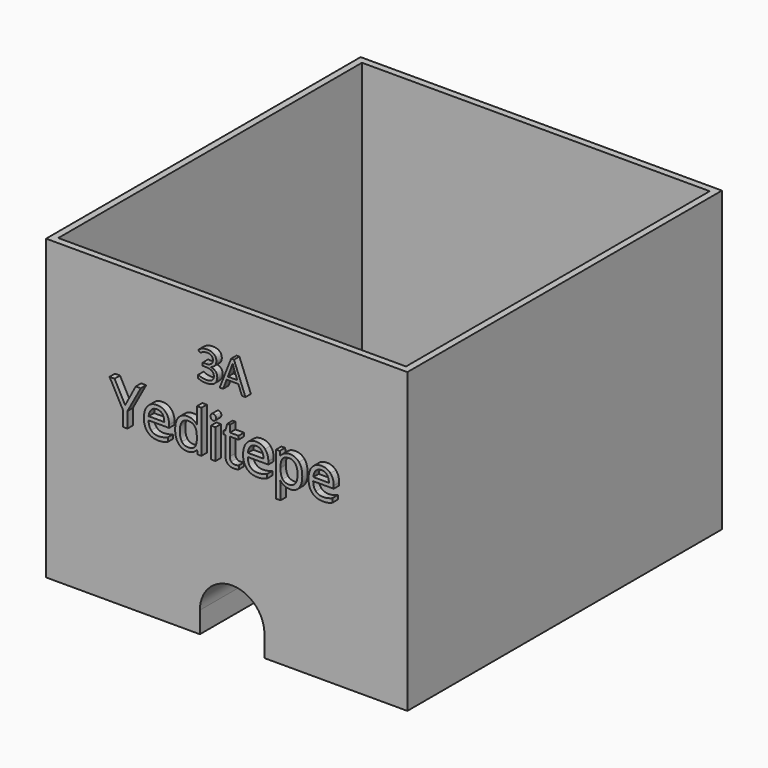
from build123d import *

# Parameters (mm, degrees)
F0_W         = 53.3
F0_H         = 44
F2_DEPTH     = 58
F3_DEPTH     = 58.001
F4_T         = -1
F5_W         = 0.6667008056
F5_H         = 4.399711482
F6_DEPTH     = 1
F7_TEXT_SIZE = 6.0143104444
F8_DEPTH     = 1


# Not quite as in the source:
# - a feature names something its author has since deleted; it is built from what else it names
# - Text() gives the source's letters only with a copy of the font that has no kerning and outlines rounded to 1/6400 em; it was checked with that copy


with BuildPart() as f2:
    # F0 (on Front) → F2 (new body)
    with BuildSketch(Plane.XZ):
        with Locations((26.65, 22)):
            Rectangle(F0_W, F0_H)
    extrude(amount=-F2_DEPTH)

    # F1 (on face) → F3 (cut, through all)
    with BuildSketch(Plane.XZ):
        with BuildLine():
            Line((22.69, 0), (27.45, 0))
            Line((27.45, 0), (32.21, 0))
            Line((32.21, 0), (32.21, 3.132))
            ThreePointArc((32.21, 3.132), (27.45, 7.892), (22.69, 3.132))
            Line((22.69, 3.132), (22.69, 0))
        make_face()
    extrude(amount=-F3_DEPTH, mode=Mode.SUBTRACT)

    # F4
    f4_openings = [f2.faces().sort_by_distance(p)[0] for p in [
        (26.65, 29, 44),
    ]]
    offset(amount=F4_T, openings=f4_openings)


with BuildPart() as f6:
    # F5 (on face) → F6 (new body)
    with BuildSketch(Plane.XZ):
        Polygon((14.0276988229, 29.7714103198), (12.4630714988, 26.836128353), (10.908720873, 29.7714103198), (10.1623756552, 29.7714103198), (12.1175175167, 26.1463049761), (12.1175175167, 23.9021309735), (12.8073408936, 23.9021309735), (12.8073408936, 26.1784196585), (14.7663365169, 29.7714103198), align=None)
        with BuildLine():
            add(Edge.make_bspline(
                [(17.3316573431, 23.8212019739), (16.3566555869, 23.8212019739), (15.7920794712, 24.4159658911)],
                knots=[0, 0, 0, 1, 1, 1], degree=2))
            add(Edge.make_bspline(
                [(18.0921330212, 23.8880005132), (17.7774091341, 23.8212019739), (17.3316573431, 23.8212019739)],
                knots=[0, 0, 0, 1, 1, 1], degree=2))
            add(Edge.make_bspline(
                [(18.760118414, 24.1063803532), (18.4068569082, 23.9547990525), (18.0921330212, 23.8880005132)],
                knots=[0, 0, 0, 1, 1, 1], degree=2))
            Line((18.760118414, 24.1063803532), (18.760118414, 24.7011442703))
            add(Edge.make_bspline(
                [(17.3560645017, 24.4044046054), (18.0664412753, 24.4044046054), (18.760118414, 24.7011442703)],
                knots=[0, 0, 0, 1, 1, 1], degree=2))
            add(Edge.make_bspline(
                [(16.3104104443, 24.8058381348), (16.6816561723, 24.4044046054), (17.3560645017, 24.4044046054)],
                knots=[0, 0, 0, 1, 1, 1], degree=2))
            add(Edge.make_bspline(
                [(15.9186113197, 25.9818778025), (15.9391647164, 25.2072716642), (16.3104104443, 24.8058381348)],
                knots=[0, 0, 0, 1, 1, 1], degree=2))
            Line((15.9186113197, 25.9818778025), (18.9489527463, 25.9818778025))
            Line((18.9489527463, 25.9818778025), (18.9489527463, 26.4032224349))
            add(Edge.make_bspline(
                [(18.467232511, 27.838748736), (18.9489527463, 27.294726017), (18.9489527463, 26.4032224349)],
                knots=[0, 0, 0, 1, 1, 1], degree=2))
            add(Edge.make_bspline(
                [(17.1595226457, 28.382771455), (17.9855122757, 28.382771455), (18.467232511, 27.838748736)],
                knots=[0, 0, 0, 1, 1, 1], degree=2))
            add(Edge.make_bspline(
                [(15.7516149715, 27.7565351492), (16.2757265874, 28.382771455), (17.1595226457, 28.382771455)],
                knots=[0, 0, 0, 1, 1, 1], degree=2))
            add(Edge.make_bspline(
                [(15.2275033555, 26.0653759766), (15.2275033555, 27.1302988433), (15.7516149715, 27.7565351492)],
                knots=[0, 0, 0, 1, 1, 1], degree=2))
            add(Edge.make_bspline(
                [(15.7920794712, 24.4159658911), (15.2275033555, 25.0107298082), (15.2275033555, 26.0653759766)],
                knots=[0, 0, 0, 1, 1, 1], degree=2))
        make_face()
        with BuildLine():
            add(Edge.make_bspline(
                [(17.1505305346, 27.8239759821), (16.6212805695, 27.8239759821), (16.3059143888, 27.4790642936)],
                knots=[0, 0, 0, 1, 1, 1], degree=2))
            add(Edge.make_bspline(
                [(17.954039887, 27.4886986984), (17.6733575633, 27.8239759821), (17.1505305346, 27.8239759821)],
                knots=[0, 0, 0, 1, 1, 1], degree=2))
            add(Edge.make_bspline(
                [(18.2347222108, 26.5239736405), (18.2347222108, 27.1534214146), (17.954039887, 27.4886986984)],
                knots=[0, 0, 0, 1, 1, 1], degree=2))
            Line((18.2347222108, 26.5239736405), (15.9340263672, 26.5239736405))
            add(Edge.make_bspline(
                [(16.3059143888, 27.4790642936), (15.9905482081, 27.1341526052), (15.9340263672, 26.5239736405)],
                knots=[0, 0, 0, 1, 1, 1], degree=2))
        make_face(mode=Mode.SUBTRACT)
        with BuildLine():
            Line((23.0442170396, 24.4917565414), (23.0801854838, 24.4917565414))
            Line((23.0801854838, 24.4917565414), (23.1688220071, 23.9021309735))
            Line((23.1688220071, 23.9021309735), (23.7109178452, 23.9021309735))
            Line((23.7109178452, 23.9021309735), (23.7109178452, 30.1490789843))
            Line((23.7109178452, 30.1490789843), (23.0442170396, 30.1490789843))
            Line((23.0442170396, 30.1490789843), (23.0442170396, 28.3583642964))
            Line((23.0442170396, 28.3583642964), (23.0609166744, 28.0487787585))
            Line((23.0609166744, 28.0487787585), (23.0891775949, 27.7314856969))
            Line((23.0891775949, 27.7314856969), (23.0365095158, 27.7314856969))
            add(Edge.make_bspline(
                [(21.6632856985, 28.382771455), (22.5586430425, 28.382771455), (23.0365095158, 27.7314856969)],
                knots=[0, 0, 0, 1, 1, 1], degree=2))
            add(Edge.make_bspline(
                [(20.3221765636, 27.7803000141), (20.8038967988, 28.382771455), (21.6632856985, 28.382771455)],
                knots=[0, 0, 0, 1, 1, 1], degree=2))
            add(Edge.make_bspline(
                [(19.8404563283, 26.0897831352), (19.8404563283, 27.1778285732), (20.3221765636, 27.7803000141)],
                knots=[0, 0, 0, 1, 1, 1], degree=2))
            add(Edge.make_bspline(
                [(20.3202496826, 24.4114698355), (19.8404563283, 25.0017376971), (19.8404563283, 26.0897831352)],
                knots=[0, 0, 0, 1, 1, 1], degree=2))
            add(Edge.make_bspline(
                [(21.6632856985, 23.8212019739), (20.8000430369, 23.8212019739), (20.3202496826, 24.4114698355)],
                knots=[0, 0, 0, 1, 1, 1], degree=2))
            add(Edge.make_bspline(
                [(23.0442170396, 24.4917565414), (22.583050201, 23.8212019739), (21.6632856985, 23.8212019739)],
                knots=[0, 0, 0, 1, 1, 1], degree=2))
        make_face()
        with BuildLine():
            add(Edge.make_bspline(
                [(21.7480684599, 24.3799974468), (22.4301843131, 24.3799974468), (22.7372006763, 24.7512431748)],
                knots=[0, 0, 0, 1, 1, 1], degree=2))
            add(Edge.make_bspline(
                [(20.8405075367, 24.8096918967), (21.1494507809, 24.3799974468), (21.7480684599, 24.3799974468)],
                knots=[0, 0, 0, 1, 1, 1], degree=2))
            add(Edge.make_bspline(
                [(20.5315642925, 26.0820756114), (20.5315642925, 25.2393863465), (20.8405075367, 24.8096918967)],
                knots=[0, 0, 0, 1, 1, 1], degree=2))
            add(Edge.make_bspline(
                [(20.8424344176, 27.3685897864), (20.5315642925, 26.9132035906), (20.5315642925, 26.0820756114)],
                knots=[0, 0, 0, 1, 1, 1], degree=2))
            add(Edge.make_bspline(
                [(21.7403609362, 27.8239759821), (21.1533045428, 27.8239759821), (20.8424344176, 27.3685897864)],
                knots=[0, 0, 0, 1, 1, 1], degree=2))
            add(Edge.make_bspline(
                [(22.7333469144, 27.4244693337), (22.4224767893, 27.8239759821), (21.7403609362, 27.8239759821)],
                knots=[0, 0, 0, 1, 1, 1], degree=2))
            add(Edge.make_bspline(
                [(23.0442170396, 26.0897831352), (23.0442170396, 27.0249626852), (22.7333469144, 27.4244693337)],
                knots=[0, 0, 0, 1, 1, 1], degree=2))
            Line((23.0442170396, 26.0897831352), (23.0442170396, 25.9497631201))
            add(Edge.make_bspline(
                [(22.7372006763, 24.7512431748), (23.0442170396, 25.1224889028), (23.0442170396, 25.9497631201)],
                knots=[0, 0, 0, 1, 1, 1], degree=2))
        make_face(mode=Mode.SUBTRACT)
        with Locations((25.4573142714, 26.1019867145)):
            Rectangle(F5_W, F5_H)
        with BuildLine():
            add(Edge.make_bspline(
                [(25.0674420277, 29.4939394643), (25.0674420277, 29.7225960026), (25.1798434159, 29.8292167481)],
                knots=[0, 0, 0, 1, 1, 1], degree=2))
            add(Edge.make_bspline(
                [(25.1798434159, 29.1586621806), (25.0674420277, 29.2691366879), (25.0674420277, 29.4939394643)],
                knots=[0, 0, 0, 1, 1, 1], degree=2))
            add(Edge.make_bspline(
                [(25.4618103269, 29.0481876733), (25.2922448041, 29.0481876733), (25.1798434159, 29.1586621806)],
                knots=[0, 0, 0, 1, 1, 1], degree=2))
            add(Edge.make_bspline(
                [(25.7386388888, 29.1586621806), (25.6223837387, 29.0481876733), (25.4618103269, 29.0481876733)],
                knots=[0, 0, 0, 1, 1, 1], degree=2))
            add(Edge.make_bspline(
                [(25.8548940389, 29.4939394643), (25.8548940389, 29.2691366879), (25.7386388888, 29.1586621806)],
                knots=[0, 0, 0, 1, 1, 1], degree=2))
            add(Edge.make_bspline(
                [(25.7386388888, 29.8272898671), (25.8548940389, 29.7187422408), (25.8548940389, 29.4939394643)],
                knots=[0, 0, 0, 1, 1, 1], degree=2))
            add(Edge.make_bspline(
                [(25.4618103269, 29.9358374935), (25.6223837387, 29.9358374935), (25.7386388888, 29.8272898671)],
                knots=[0, 0, 0, 1, 1, 1], degree=2))
            add(Edge.make_bspline(
                [(25.1798434159, 29.8292167481), (25.2922448041, 29.9358374935), (25.4618103269, 29.9358374935)],
                knots=[0, 0, 0, 1, 1, 1], degree=2))
        make_face()
        with BuildLine():
            Line((26.9984875229, 28.2710156541), (27.0092743154, 27.784153776))
            Line((27.0092743154, 27.784153776), (27.2525250148, 27.784153776))
            Line((27.2525250148, 27.784153776), (27.2525250148, 25.1661648708))
            add(Edge.make_bspline(
                [(28.5281201978, 23.8212019739), (27.2525250148, 23.8212019739), (27.2525250148, 25.1661648708)],
                knots=[0, 0, 0, 1, 1, 1], degree=2))
            add(Edge.make_bspline(
                [(28.9083580368, 23.8558858309), (28.6976857206, 23.8212019739), (28.5281201978, 23.8212019739)],
                knots=[0, 0, 0, 1, 1, 1], degree=2))
            add(Edge.make_bspline(
                [(29.2269356857, 23.9419531796), (29.119030353, 23.8905696878), (28.9083580368, 23.8558858309)],
                knots=[0, 0, 0, 1, 1, 1], degree=2))
            Line((29.2269356857, 23.9419531796), (29.2269356857, 24.4519343353))
            add(Edge.make_bspline(
                [(28.966164465, 24.3979816689), (29.1305916387, 24.4236734148), (29.2269356857, 24.4519343353)],
                knots=[0, 0, 0, 1, 1, 1], degree=2))
            add(Edge.make_bspline(
                [(28.6244642448, 24.3722899231), (28.8017372914, 24.3722899231), (28.966164465, 24.3979816689)],
                knots=[0, 0, 0, 1, 1, 1], degree=2))
            add(Edge.make_bspline(
                [(28.1067755653, 24.5848891202), (28.2956098975, 24.3722899231), (28.6244642448, 24.3722899231)],
                knots=[0, 0, 0, 1, 1, 1], degree=2))
            add(Edge.make_bspline(
                [(27.9179412331, 25.1944257912), (27.9179412331, 24.7974883174), (28.1067755653, 24.5848891202)],
                knots=[0, 0, 0, 1, 1, 1], degree=2))
            Line((27.9179412331, 25.1944257912), (27.9179412331, 27.784153776))
            Line((27.9179412331, 27.784153776), (29.1948210034, 27.784153776))
            Line((29.1948210034, 27.784153776), (29.1948210034, 28.3018424555))
            Line((29.1948210034, 28.3018424555), (27.9179412331, 28.3018424555))
            Line((27.9179412331, 28.3018424555), (27.9179412331, 29.3218047669))
            Line((27.9179412331, 29.3218047669), (27.5325650449, 29.3218047669))
            Line((27.5325650449, 29.3218047669), (27.2525250148, 28.382771455))
            Line((27.2525250148, 28.382771455), (26.9984875229, 28.2710156541))
        make_face()
        with BuildLine():
            add(Edge.make_bspline(
                [(31.9643912093, 23.8212019739), (30.9893894531, 23.8212019739), (30.4248133374, 24.4159658911)],
                knots=[0, 0, 0, 1, 1, 1], degree=2))
            add(Edge.make_bspline(
                [(32.7248668873, 23.8880005132), (32.4101430003, 23.8212019739), (31.9643912093, 23.8212019739)],
                knots=[0, 0, 0, 1, 1, 1], degree=2))
            add(Edge.make_bspline(
                [(33.3928522802, 24.1063803532), (33.0395907744, 23.9547990525), (32.7248668873, 23.8880005132)],
                knots=[0, 0, 0, 1, 1, 1], degree=2))
            Line((33.3928522802, 24.1063803532), (33.3928522802, 24.7011442703))
            add(Edge.make_bspline(
                [(31.9887983678, 24.4044046054), (32.6991751414, 24.4044046054), (33.3928522802, 24.7011442703)],
                knots=[0, 0, 0, 1, 1, 1], degree=2))
            add(Edge.make_bspline(
                [(30.9431443105, 24.8058381348), (31.3143900385, 24.4044046054), (31.9887983678, 24.4044046054)],
                knots=[0, 0, 0, 1, 1, 1], degree=2))
            add(Edge.make_bspline(
                [(30.5513451858, 25.9818778025), (30.5718985825, 25.2072716642), (30.9431443105, 24.8058381348)],
                knots=[0, 0, 0, 1, 1, 1], degree=2))
            Line((30.5513451858, 25.9818778025), (33.5816866124, 25.9818778025))
            Line((33.5816866124, 25.9818778025), (33.5816866124, 26.4032224349))
            add(Edge.make_bspline(
                [(33.0999663772, 27.838748736), (33.5816866124, 27.294726017), (33.5816866124, 26.4032224349)],
                knots=[0, 0, 0, 1, 1, 1], degree=2))
            add(Edge.make_bspline(
                [(31.7922565119, 28.382771455), (32.6182461419, 28.382771455), (33.0999663772, 27.838748736)],
                knots=[0, 0, 0, 1, 1, 1], degree=2))
            add(Edge.make_bspline(
                [(30.3843488376, 27.7565351492), (30.9084604536, 28.382771455), (31.7922565119, 28.382771455)],
                knots=[0, 0, 0, 1, 1, 1], degree=2))
            add(Edge.make_bspline(
                [(29.8602372217, 26.0653759766), (29.8602372217, 27.1302988433), (30.3843488376, 27.7565351492)],
                knots=[0, 0, 0, 1, 1, 1], degree=2))
            add(Edge.make_bspline(
                [(30.4248133374, 24.4159658911), (29.8602372217, 25.0107298082), (29.8602372217, 26.0653759766)],
                knots=[0, 0, 0, 1, 1, 1], degree=2))
        make_face()
        with BuildLine():
            add(Edge.make_bspline(
                [(31.7832644008, 27.8239759821), (31.2540144357, 27.8239759821), (30.938648255, 27.4790642936)],
                knots=[0, 0, 0, 1, 1, 1], degree=2))
            add(Edge.make_bspline(
                [(32.5867737532, 27.4886986984), (32.3060914295, 27.8239759821), (31.7832644008, 27.8239759821)],
                knots=[0, 0, 0, 1, 1, 1], degree=2))
            add(Edge.make_bspline(
                [(32.867456077, 26.5239736405), (32.867456077, 27.1534214146), (32.5867737532, 27.4886986984)],
                knots=[0, 0, 0, 1, 1, 1], degree=2))
            Line((32.867456077, 26.5239736405), (30.5667602334, 26.5239736405))
            add(Edge.make_bspline(
                [(30.938648255, 27.4790642936), (30.6232820743, 27.1341526052), (30.5667602334, 26.5239736405)],
                knots=[0, 0, 0, 1, 1, 1], degree=2))
        make_face(mode=Mode.SUBTRACT)
        with BuildLine():
            add(Edge.make_bspline(
                [(36.7661785143, 23.8212019739), (36.3358417708, 23.8212019739), (35.980653384, 23.9798485047)],
                knots=[0, 0, 0, 1, 1, 1], degree=2))
            add(Edge.make_bspline(
                [(38.1092145302, 24.4217465339), (37.625567414, 23.8212019739), (36.7661785143, 23.8212019739)],
                knots=[0, 0, 0, 1, 1, 1], degree=2))
            add(Edge.make_bspline(
                [(38.5928616464, 26.10648277), (38.5928616464, 25.0222910938), (38.1092145302, 24.4217465339)],
                knots=[0, 0, 0, 1, 1, 1], degree=2))
            add(Edge.make_bspline(
                [(38.116922054, 27.784153776), (38.5928616464, 27.185536097), (38.5928616464, 26.10648277)],
                knots=[0, 0, 0, 1, 1, 1], degree=2))
            add(Edge.make_bspline(
                [(36.7661785143, 28.382771455), (37.6409824615, 28.382771455), (38.116922054, 27.784153776)],
                knots=[0, 0, 0, 1, 1, 1], degree=2))
            add(Edge.make_bspline(
                [(35.9832225586, 28.2221980432), (36.3242804852, 28.382771455), (36.7661785143, 28.382771455)],
                knots=[0, 0, 0, 1, 1, 1], degree=2))
            add(Edge.make_bspline(
                [(35.3852471732, 27.6993710146), (35.642164632, 28.0616246315), (35.9832225586, 28.2221980432)],
                knots=[0, 0, 0, 1, 1, 1], degree=2))
            Line((35.3852471732, 27.6993710146), (35.3531324909, 27.6993710146))
            Line((35.3531324909, 27.6993710146), (35.2606422057, 28.3018424555))
            Line((35.2606422057, 28.3018424555), (34.7185463676, 28.3018424555))
            Line((34.7185463676, 28.3018424555), (34.7185463676, 21.9264357153))
            Line((34.7185463676, 21.9264357153), (35.3852471732, 21.9264357153))
            Line((35.3852471732, 21.9264357153), (35.3852471732, 23.7377037998))
            add(Edge.make_bspline(
                [(35.3364328561, 24.4686339701), (35.3852471732, 24.0832577819), (35.3852471732, 23.7377037998)],
                knots=[0, 0, 0, 1, 1, 1], degree=2))
            Line((35.3364328561, 24.4686339701), (35.3852471732, 24.4686339701))
            add(Edge.make_bspline(
                [(35.980653384, 23.9798485047), (35.6254649972, 24.1384950356), (35.3852471732, 24.4686339701)],
                knots=[0, 0, 0, 1, 1, 1], degree=2))
        make_face()
        with BuildLine():
            add(Edge.make_bspline(
                [(36.6698344672, 27.8162684583), (35.9954261379, 27.8162684583), (35.6941904174, 27.4430958494)],
                knots=[0, 0, 0, 1, 1, 1], degree=2))
            add(Edge.make_bspline(
                [(37.5786799778, 27.3769396038), (37.2556062733, 27.8162684583), (36.6698344672, 27.8162684583)],
                knots=[0, 0, 0, 1, 1, 1], degree=2))
            add(Edge.make_bspline(
                [(37.9017536822, 26.1141902938), (37.9017536822, 26.9376107492), (37.5786799778, 27.3769396038)],
                knots=[0, 0, 0, 1, 1, 1], degree=2))
            add(Edge.make_bspline(
                [(37.5786799778, 24.841806579), (37.9017536822, 25.3036157112), (37.9017536822, 26.1141902938)],
                knots=[0, 0, 0, 1, 1, 1], degree=2))
            add(Edge.make_bspline(
                [(36.6852495148, 24.3799974468), (37.2556062733, 24.3799974468), (37.5786799778, 24.841806579)],
                knots=[0, 0, 0, 1, 1, 1], degree=2))
            add(Edge.make_bspline(
                [(35.6941904174, 24.7795040953), (36.0031336617, 24.3799974468), (36.6852495148, 24.3799974468)],
                knots=[0, 0, 0, 1, 1, 1], degree=2))
            add(Edge.make_bspline(
                [(35.3852471732, 26.10648277), (35.3852471732, 25.1790107437), (35.6941904174, 24.7795040953)],
                knots=[0, 0, 0, 1, 1, 1], degree=2))
            Line((35.3852471732, 26.10648277), (35.3852471732, 26.2542103088))
            add(Edge.make_bspline(
                [(35.6941904174, 27.4430958494), (35.392954697, 27.0699232405), (35.3852471732, 26.2542103088)],
                knots=[0, 0, 0, 1, 1, 1], degree=2))
        make_face(mode=Mode.SUBTRACT)
        with BuildLine():
            add(Edge.make_bspline(
                [(41.6154955492, 23.8212019739), (40.6404937931, 23.8212019739), (40.0759176773, 24.4159658911)],
                knots=[0, 0, 0, 1, 1, 1], degree=2))
            add(Edge.make_bspline(
                [(42.3759712273, 23.8880005132), (42.0612473402, 23.8212019739), (41.6154955492, 23.8212019739)],
                knots=[0, 0, 0, 1, 1, 1], degree=2))
            add(Edge.make_bspline(
                [(43.0439566202, 24.1063803532), (42.6906951143, 23.9547990525), (42.3759712273, 23.8880005132)],
                knots=[0, 0, 0, 1, 1, 1], degree=2))
            Line((43.0439566202, 24.1063803532), (43.0439566202, 24.7011442703))
            add(Edge.make_bspline(
                [(41.6399027078, 24.4044046054), (42.3502794814, 24.4044046054), (43.0439566202, 24.7011442703)],
                knots=[0, 0, 0, 1, 1, 1], degree=2))
            add(Edge.make_bspline(
                [(40.5942486505, 24.8058381348), (40.9654943784, 24.4044046054), (41.6399027078, 24.4044046054)],
                knots=[0, 0, 0, 1, 1, 1], degree=2))
            add(Edge.make_bspline(
                [(40.2024495258, 25.9818778025), (40.2230029225, 25.2072716642), (40.5942486505, 24.8058381348)],
                knots=[0, 0, 0, 1, 1, 1], degree=2))
            Line((40.2024495258, 25.9818778025), (43.2327909524, 25.9818778025))
            Line((43.2327909524, 25.9818778025), (43.2327909524, 26.4032224349))
            add(Edge.make_bspline(
                [(42.7510707171, 27.838748736), (43.2327909524, 27.294726017), (43.2327909524, 26.4032224349)],
                knots=[0, 0, 0, 1, 1, 1], degree=2))
            add(Edge.make_bspline(
                [(41.4433608518, 28.382771455), (42.2693504819, 28.382771455), (42.7510707171, 27.838748736)],
                knots=[0, 0, 0, 1, 1, 1], degree=2))
            add(Edge.make_bspline(
                [(40.0354531776, 27.7565351492), (40.5595647935, 28.382771455), (41.4433608518, 28.382771455)],
                knots=[0, 0, 0, 1, 1, 1], degree=2))
            add(Edge.make_bspline(
                [(39.5113415616, 26.0653759766), (39.5113415616, 27.1302988433), (40.0354531776, 27.7565351492)],
                knots=[0, 0, 0, 1, 1, 1], degree=2))
            add(Edge.make_bspline(
                [(40.0759176773, 24.4159658911), (39.5113415616, 25.0107298082), (39.5113415616, 26.0653759766)],
                knots=[0, 0, 0, 1, 1, 1], degree=2))
        make_face()
        with BuildLine():
            add(Edge.make_bspline(
                [(41.4343687408, 27.8239759821), (40.9051187756, 27.8239759821), (40.5897525949, 27.4790642936)],
                knots=[0, 0, 0, 1, 1, 1], degree=2))
            add(Edge.make_bspline(
                [(42.2378780932, 27.4886986984), (41.9571957694, 27.8239759821), (41.4343687408, 27.8239759821)],
                knots=[0, 0, 0, 1, 1, 1], degree=2))
            add(Edge.make_bspline(
                [(42.5185604169, 26.5239736405), (42.5185604169, 27.1534214146), (42.2378780932, 27.4886986984)],
                knots=[0, 0, 0, 1, 1, 1], degree=2))
            Line((42.5185604169, 26.5239736405), (40.2178645733, 26.5239736405))
            add(Edge.make_bspline(
                [(40.5897525949, 27.4790642936), (40.2743864143, 27.1341526052), (40.2178645733, 26.5239736405)],
                knots=[0, 0, 0, 1, 1, 1], degree=2))
        make_face(mode=Mode.SUBTRACT)
    extrude(amount=F6_DEPTH)


with BuildPart() as f8:
    # F7 (on face) → F8 (new body)
    with BuildSketch(Plane.XZ):
        with Locations((22.9661621848, 33.6500485252)):
            Text('3A', F7_TEXT_SIZE, font='Open Sans', text_align=(TextAlign.LEFT, TextAlign.BOTTOM))
    extrude(amount=F8_DEPTH)


solid = Compound([f2.part, f6.part, f8.part])
